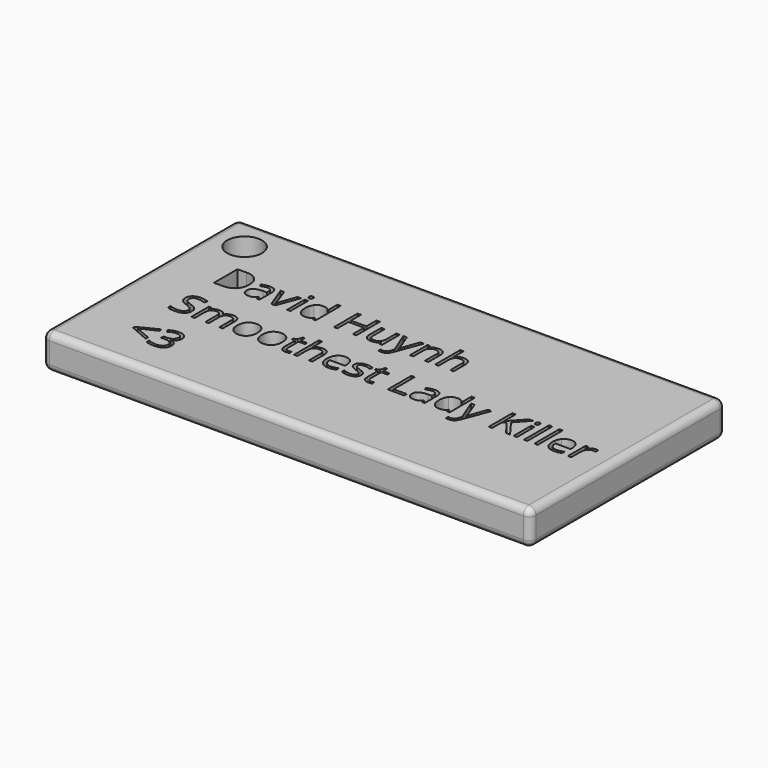
from build123d import *

# Parameters (mm, degrees)
F0_W     = 70
F0_H     = 35
F0_W_2   = 0.4794088215
F0_H_2   = 3.1637287353
F0_H_3   = 4.4920329459
F0_R     = 2.5
F1_DEPTH = 5
F2_R     = 1


with BuildPart() as f1:
    # F0 (on Top) → F1 (new body)
    with BuildSketch(Plane.XY):
        with Locations((35, 17.5)):
            Rectangle(F0_W, F0_H)
        Polygon((10.2831517034, 6.0801306554), (10.2831517034, 5.6441365056), (7.5092312969, 6.8625184624), (7.5092312969, 7.1451756866), (10.2831517034, 8.5279791659), (10.2831517034, 8.0984510311), (8.0255887752, 7.026939985), align=None, mode=Mode.SUBTRACT)
        with BuildLine():
            add(Edge.make_bspline(
                [(13.152214901, 8.9450371291), (13.4930662596, 8.6637654795), (13.4930662596, 8.173272061)],
                knots=[0, 0, 0, 1, 1, 1], degree=2))
            add(Edge.make_bspline(
                [(13.4930662596, 8.173272061), (13.4930662596, 7.7686842695), (13.2662938787, 7.511891105)],
                knots=[0, 0, 0, 1, 1, 1], degree=2))
            add(Edge.make_bspline(
                [(13.2662938787, 7.511891105), (13.0395214978, 7.2550979405), (12.6238491093, 7.1682685971)],
                knots=[0, 0, 0, 1, 1, 1], degree=2))
            Line((12.6238491093, 7.1682685971), (12.6238491093, 7.1451756866))
            add(Edge.make_bspline(
                [(12.6238491093, 7.1451756866), (13.1318931398, 7.0823629701), (13.377139849, 6.8223367981)],
                knots=[0, 0, 0, 1, 1, 1], degree=2))
            add(Edge.make_bspline(
                [(13.377139849, 6.8223367981), (13.6223865583, 6.5623106262), (13.6223865583, 6.1410959391)],
                knots=[0, 0, 0, 1, 1, 1], degree=2))
            add(Edge.make_bspline(
                [(13.6223865583, 6.1410959391), (13.6223865583, 5.5379091174), (13.2039430204, 5.2127609379)],
                knots=[0, 0, 0, 1, 1, 1], degree=2))
            add(Edge.make_bspline(
                [(13.2039430204, 5.2127609379), (12.7854994826, 4.8876127584), (12.0151199891, 4.8876127584)],
                knots=[0, 0, 0, 1, 1, 1], degree=2))
            add(Edge.make_bspline(
                [(12.0151199891, 4.8876127584), (11.679810929, 4.8876127584), (11.4013104286, 4.9384171615)],
                knots=[0, 0, 0, 1, 1, 1], degree=2))
            add(Edge.make_bspline(
                [(11.4013104286, 4.9384171615), (11.1228099283, 4.9892215645), (10.8604744653, 5.1157707139)],
                knots=[0, 0, 0, 1, 1, 1], degree=2))
            Line((10.8604744653, 5.1157707139), (10.8604744653, 5.5720866249))
            add(Edge.make_bspline(
                [(10.8604744653, 5.5720866249), (11.1348182417, 5.4363003113), (11.4451869586, 5.3656360053)],
                knots=[0, 0, 0, 1, 1, 1], degree=2))
            add(Edge.make_bspline(
                [(11.4451869586, 5.3656360053), (11.7555556754, 5.2949716992), (12.0326706011, 5.2949716992)],
                knots=[0, 0, 0, 1, 1, 1], degree=2))
            add(Edge.make_bspline(
                [(12.0326706011, 5.2949716992), (13.1263508412, 5.2949716992), (13.1263508412, 6.1521805361)],
                knots=[0, 0, 0, 1, 1, 1], degree=2))
            add(Edge.make_bspline(
                [(13.1263508412, 6.1521805361), (13.1263508412, 6.9207125968), (11.9199771979, 6.9207125968)],
                knots=[0, 0, 0, 1, 1, 1], degree=2))
            Line((11.9199771979, 6.9207125968), (11.5043048094, 6.9207125968))
            Line((11.5043048094, 6.9207125968), (11.5043048094, 7.3326901197))
            Line((11.5043048094, 7.3326901197), (11.9255194965, 7.3326901197))
            add(Edge.make_bspline(
                [(11.9255194965, 7.3326901197), (12.4187840642, 7.3326901197), (12.7074454452, 7.5506871946)],
                knots=[0, 0, 0, 1, 1, 1], degree=2))
            add(Edge.make_bspline(
                [(12.7074454452, 7.5506871946), (12.9961068262, 7.7686842695), (12.9961068262, 8.1557214491)],
                knots=[0, 0, 0, 1, 1, 1], degree=2))
            add(Edge.make_bspline(
                [(12.9961068262, 8.1557214491), (12.9961068262, 8.464242733), (12.784113908, 8.6406725691)],
                knots=[0, 0, 0, 1, 1, 1], degree=2))
            add(Edge.make_bspline(
                [(12.784113908, 8.6406725691), (12.5721209898, 8.8171024051), (12.2081767207, 8.8171024051)],
                knots=[0, 0, 0, 1, 1, 1], degree=2))
            add(Edge.make_bspline(
                [(12.2081767207, 8.8171024051), (11.931061795, 8.8171024051), (11.6858150857, 8.7418195169)],
                knots=[0, 0, 0, 1, 1, 1], degree=2))
            add(Edge.make_bspline(
                [(11.6858150857, 8.7418195169), (11.4405683765, 8.6665366288), (11.1255810776, 8.464242733)],
                knots=[0, 0, 0, 1, 1, 1], degree=2))
            Line((11.1255810776, 8.464242733), (10.8835673758, 8.7875434797))
            add(Edge.make_bspline(
                [(10.8835673758, 8.7875434797), (11.1431316895, 8.9926085247), (11.4821356153, 9.1094586517)],
                knots=[0, 0, 0, 1, 1, 1], degree=2))
            add(Edge.make_bspline(
                [(11.4821356153, 9.1094586517), (11.8211395411, 9.2263087787), (12.1970921237, 9.2263087787)],
                knots=[0, 0, 0, 1, 1, 1], degree=2))
            add(Edge.make_bspline(
                [(12.1970921237, 9.2263087787), (12.8113635423, 9.2263087787), (13.152214901, 8.9450371291)],
                knots=[0, 0, 0, 1, 1, 1], degree=2))
        make_face(mode=Mode.SUBTRACT)
        with BuildLine():
            add(Edge.make_bspline(
                [(9.9210548671, 14.8129456812), (10.1704583003, 14.541373054), (10.1704583003, 14.1090737699)],
                knots=[0, 0, 0, 1, 1, 1], degree=2))
            add(Edge.make_bspline(
                [(10.1704583003, 14.1090737699), (10.1704583003, 13.5520727692), (9.7663323669, 13.2398566196)],
                knots=[0, 0, 0, 1, 1, 1], degree=2))
            add(Edge.make_bspline(
                [(9.7663323669, 13.2398566196), (9.3622064336, 12.9276404699), (8.6694191193, 12.9276404699)],
                knots=[0, 0, 0, 1, 1, 1], degree=2))
            add(Edge.make_bspline(
                [(8.6694191193, 12.9276404699), (7.919361387, 12.9276404699), (7.5147735955, 13.1216209179)],
                knots=[0, 0, 0, 1, 1, 1], degree=2))
            Line((7.5147735955, 13.1216209179), (7.5147735955, 13.5945637245))
            add(Edge.make_bspline(
                [(7.5147735955, 13.5945637245), (7.7752616256, 13.485565187), (8.0810117603, 13.4218287541)],
                knots=[0, 0, 0, 1, 1, 1], degree=2))
            add(Edge.make_bspline(
                [(8.0810117603, 13.4218287541), (8.386761895, 13.3580923212), (8.6869697312, 13.3580923212)],
                knots=[0, 0, 0, 1, 1, 1], degree=2))
            add(Edge.make_bspline(
                [(8.6869697312, 13.3580923212), (9.1774631498, 13.3580923212), (9.4259428665, 13.5442211796)],
                knots=[0, 0, 0, 1, 1, 1], degree=2))
            add(Edge.make_bspline(
                [(9.4259428665, 13.5442211796), (9.6744225832, 13.7303500381), (9.6744225832, 14.0628879489)],
                knots=[0, 0, 0, 1, 1, 1], degree=2))
            add(Edge.make_bspline(
                [(9.6744225832, 14.0628879489), (9.6744225832, 14.2818087403), (9.5862076652, 14.4217517777)],
                knots=[0, 0, 0, 1, 1, 1], degree=2))
            add(Edge.make_bspline(
                [(9.5862076652, 14.4217517777), (9.4979927472, 14.5616948152), (9.2915421275, 14.6803923751)],
                knots=[0, 0, 0, 1, 1, 1], degree=2))
            add(Edge.make_bspline(
                [(9.2915421275, 14.6803923751), (9.0850915079, 14.7990899349), (8.6638768208, 14.9487319948)],
                knots=[0, 0, 0, 1, 1, 1], degree=2))
            add(Edge.make_bspline(
                [(8.6638768208, 14.9487319948), (8.0754694618, 15.1593393384), (7.8228330212, 15.4480007193)],
                knots=[0, 0, 0, 1, 1, 1], degree=2))
            add(Edge.make_bspline(
                [(7.8228330212, 15.4480007193), (7.5701965806, 15.7366621003), (7.5701965806, 16.2012914591)],
                knots=[0, 0, 0, 1, 1, 1], degree=2))
            add(Edge.make_bspline(
                [(7.5701965806, 16.2012914591), (7.5701965806, 16.6890137283), (7.9364501408, 16.9776751093)],
                knots=[0, 0, 0, 1, 1, 1], degree=2))
            add(Edge.make_bspline(
                [(7.9364501408, 16.9776751093), (8.3027037009, 17.2663364902), (8.906814239, 17.2663364902)],
                knots=[0, 0, 0, 1, 1, 1], degree=2))
            add(Edge.make_bspline(
                [(8.906814239, 17.2663364902), (9.5358651204, 17.2663364902), (10.0642309121, 17.0354073855)],
                knots=[0, 0, 0, 1, 1, 1], degree=2))
            Line((10.0642309121, 17.0354073855), (9.9108939865, 16.6086503999))
            add(Edge.make_bspline(
                [(9.9108939865, 16.6086503999), (9.3880704933, 16.8275711912), (8.8948059255, 16.8275711912)],
                knots=[0, 0, 0, 1, 1, 1], degree=2))
            add(Edge.make_bspline(
                [(8.8948059255, 16.8275711912), (8.5049975967, 16.8275711912), (8.2856149472, 16.6603785193)],
                knots=[0, 0, 0, 1, 1, 1], degree=2))
            add(Edge.make_bspline(
                [(8.2856149472, 16.6603785193), (8.0662322976, 16.4931858475), (8.0662322976, 16.1957491605)],
                knots=[0, 0, 0, 1, 1, 1], degree=2))
            add(Edge.make_bspline(
                [(8.0662322976, 16.1957491605), (8.0662322976, 15.9768283692), (8.1470574843, 15.8364234735)],
                knots=[0, 0, 0, 1, 1, 1], degree=2))
            add(Edge.make_bspline(
                [(8.1470574843, 15.8364234735), (8.227882671, 15.6960185778), (8.4200156861, 15.5791684508)],
                knots=[0, 0, 0, 1, 1, 1], degree=2))
            add(Edge.make_bspline(
                [(8.4200156861, 15.5791684508), (8.6121487013, 15.4623183238), (9.0074993287, 15.3209897117)],
                knots=[0, 0, 0, 1, 1, 1], degree=2))
            add(Edge.make_bspline(
                [(9.0074993287, 15.3209897117), (9.671651434, 15.0845183084), (9.9210548671, 14.8129456812)],
                knots=[0, 0, 0, 1, 1, 1], degree=2))
        make_face(mode=Mode.SUBTRACT)
        with BuildLine():
            Line((15.4735142621, 12.9858346043), (14.995029157, 12.9858346043))
            Line((14.995029157, 12.9858346043), (14.995029157, 15.043874786))
            add(Edge.make_bspline(
                [(14.995029157, 15.043874786), (14.995029157, 15.4225985178), (14.8333787837, 15.6114985255)],
                knots=[0, 0, 0, 1, 1, 1], degree=2))
            add(Edge.make_bspline(
                [(14.8333787837, 15.6114985255), (14.6717284103, 15.8003985332), (14.3308770517, 15.8003985332)],
                knots=[0, 0, 0, 1, 1, 1], degree=2))
            add(Edge.make_bspline(
                [(14.3308770517, 15.8003985332), (13.8837983049, 15.8003985332), (13.6699579539, 15.5436053687)],
                knots=[0, 0, 0, 1, 1, 1], degree=2))
            add(Edge.make_bspline(
                [(13.6699579539, 15.5436053687), (13.4561176028, 15.2868122042), (13.4561176028, 14.752904114)],
                knots=[0, 0, 0, 1, 1, 1], degree=2))
            Line((13.4561176028, 14.752904114), (13.4561176028, 12.9858346043))
            Line((13.4561176028, 12.9858346043), (12.9767087814, 12.9858346043))
            Line((12.9767087814, 12.9858346043), (12.9767087814, 15.043874786))
            add(Edge.make_bspline(
                [(12.9767087814, 15.043874786), (12.9767087814, 15.4225985178), (12.815058408, 15.6114985255)],
                knots=[0, 0, 0, 1, 1, 1], degree=2))
            add(Edge.make_bspline(
                [(12.815058408, 15.6114985255), (12.6534080347, 15.8003985332), (12.3097855268, 15.8003985332)],
                knots=[0, 0, 0, 1, 1, 1], degree=2))
            add(Edge.make_bspline(
                [(12.3097855268, 15.8003985332), (11.8599356307, 15.8003985332), (11.6507138618, 15.5306733388)],
                knots=[0, 0, 0, 1, 1, 1], degree=2))
            add(Edge.make_bspline(
                [(11.6507138618, 15.5306733388), (11.4414920929, 15.2609481445), (11.4414920929, 14.6457530094)],
                knots=[0, 0, 0, 1, 1, 1], degree=2))
            Line((11.4414920929, 14.6457530094), (11.4414920929, 12.9858346043))
            Line((11.4414920929, 12.9858346043), (10.9620832714, 12.9858346043))
            Line((10.9620832714, 12.9858346043), (10.9620832714, 16.1495633396))
            Line((10.9620832714, 16.1495633396), (11.3518916002, 16.1495633396))
            Line((11.3518916002, 16.1495633396), (11.4294837794, 15.7163403391))
            Line((11.4294837794, 15.7163403391), (11.4525766899, 15.7163403391))
            add(Edge.make_bspline(
                [(11.4525766899, 15.7163403391), (11.5883630035, 15.9472694438), (11.8354571456, 16.0775134589)],
                knots=[0, 0, 0, 1, 1, 1], degree=2))
            add(Edge.make_bspline(
                [(11.8354571456, 16.0775134589), (12.0825512877, 16.207757474), (12.3883014224, 16.207757474)],
                knots=[0, 0, 0, 1, 1, 1], degree=2))
            add(Edge.make_bspline(
                [(12.3883014224, 16.207757474), (13.1300457069, 16.207757474), (13.3582036624, 15.6701545181)],
                knots=[0, 0, 0, 1, 1, 1], degree=2))
            Line((13.3582036624, 15.6701545181), (13.3812965729, 15.6701545181))
            add(Edge.make_bspline(
                [(13.3812965729, 15.6701545181), (13.522625185, 15.9186342348), (13.7909648048, 16.0631958544)],
                knots=[0, 0, 0, 1, 1, 1], degree=2))
            add(Edge.make_bspline(
                [(13.7909648048, 16.0631958544), (14.0593044245, 16.207757474), (14.4029269324, 16.207757474)],
                knots=[0, 0, 0, 1, 1, 1], degree=2))
            add(Edge.make_bspline(
                [(14.4029269324, 16.207757474), (14.9396061719, 16.207757474), (15.206560217, 15.9320281229)],
                knots=[0, 0, 0, 1, 1, 1], degree=2))
            add(Edge.make_bspline(
                [(15.206560217, 15.9320281229), (15.4735142621, 15.6562987718), (15.4735142621, 15.0494170845)],
                knots=[0, 0, 0, 1, 1, 1], degree=2))
            Line((15.4735142621, 15.0494170845), (15.4735142621, 12.9858346043))
        make_face(mode=Mode.SUBTRACT)
        with BuildLine():
            add(Edge.make_bspline(
                [(18.8002789453, 15.7657591675), (19.1914728488, 15.323760861), (19.1914728488, 14.5709319794)],
                knots=[0, 0, 0, 1, 1, 1], degree=2))
            add(Edge.make_bspline(
                [(19.1914728488, 14.5709319794), (19.1914728488, 13.7968576202), (18.8021263782, 13.3622490451)],
                knots=[0, 0, 0, 1, 1, 1], degree=2))
            add(Edge.make_bspline(
                [(18.8021263782, 13.3622490451), (18.4127799075, 12.9276404699), (17.7255348917, 12.9276404699)],
                knots=[0, 0, 0, 1, 1, 1], degree=2))
            add(Edge.make_bspline(
                [(17.7255348917, 12.9276404699), (17.300625339, 12.9276404699), (16.9717822938, 13.1271632164)],
                knots=[0, 0, 0, 1, 1, 1], degree=2))
            add(Edge.make_bspline(
                [(16.9717822938, 13.1271632164), (16.6429392486, 13.3266859629), (16.4637382633, 13.6989436798)],
                knots=[0, 0, 0, 1, 1, 1], degree=2))
            add(Edge.make_bspline(
                [(16.4637382633, 13.6989436798), (16.284537278, 14.0712013967), (16.284537278, 14.5709319794)],
                knots=[0, 0, 0, 1, 1, 1], degree=2))
            add(Edge.make_bspline(
                [(16.284537278, 14.5709319794), (16.284537278, 15.3440826222), (16.6715744576, 15.7759200481)],
                knots=[0, 0, 0, 1, 1, 1], degree=2))
            add(Edge.make_bspline(
                [(16.6715744576, 15.7759200481), (17.0586116372, 16.207757474), (17.745856653, 16.207757474)],
                knots=[0, 0, 0, 1, 1, 1], degree=2))
            add(Edge.make_bspline(
                [(17.745856653, 16.207757474), (18.4090850418, 16.207757474), (18.8002789453, 15.7657591675)],
                knots=[0, 0, 0, 1, 1, 1], degree=2))
        make_face(mode=Mode.SUBTRACT)
        with BuildLine():
            add(Edge.make_bspline(
                [(22.3713666214, 15.7657591675), (22.7625605249, 15.323760861), (22.7625605249, 14.5709319794)],
                knots=[0, 0, 0, 1, 1, 1], degree=2))
            add(Edge.make_bspline(
                [(22.7625605249, 14.5709319794), (22.7625605249, 13.7968576202), (22.3732140542, 13.3622490451)],
                knots=[0, 0, 0, 1, 1, 1], degree=2))
            add(Edge.make_bspline(
                [(22.3732140542, 13.3622490451), (21.9838675836, 12.9276404699), (21.2966225678, 12.9276404699)],
                knots=[0, 0, 0, 1, 1, 1], degree=2))
            add(Edge.make_bspline(
                [(21.2966225678, 12.9276404699), (20.8717130151, 12.9276404699), (20.5428699699, 13.1271632164)],
                knots=[0, 0, 0, 1, 1, 1], degree=2))
            add(Edge.make_bspline(
                [(20.5428699699, 13.1271632164), (20.2140269247, 13.3266859629), (20.0348259394, 13.6989436798)],
                knots=[0, 0, 0, 1, 1, 1], degree=2))
            add(Edge.make_bspline(
                [(20.0348259394, 13.6989436798), (19.8556249541, 14.0712013967), (19.8556249541, 14.5709319794)],
                knots=[0, 0, 0, 1, 1, 1], degree=2))
            add(Edge.make_bspline(
                [(19.8556249541, 14.5709319794), (19.8556249541, 15.3440826222), (20.2426621337, 15.7759200481)],
                knots=[0, 0, 0, 1, 1, 1], degree=2))
            add(Edge.make_bspline(
                [(20.2426621337, 15.7759200481), (20.6296993133, 16.207757474), (21.316944329, 16.207757474)],
                knots=[0, 0, 0, 1, 1, 1], degree=2))
            add(Edge.make_bspline(
                [(21.316944329, 16.207757474), (21.9801727179, 16.207757474), (22.3713666214, 15.7657591675)],
                knots=[0, 0, 0, 1, 1, 1], degree=2))
        make_face(mode=Mode.SUBTRACT)
        with BuildLine():
            add(Edge.make_bspline(
                [(24.2525151088, 13.476789881), (24.3883014224, 13.3239148137), (24.6247728257, 13.3239148137)],
                knots=[0, 0, 0, 1, 1, 1], degree=2))
            add(Edge.make_bspline(
                [(24.6247728257, 13.3239148137), (24.7522456915, 13.3239148137), (24.8704813932, 13.3423891421)],
                knots=[0, 0, 0, 1, 1, 1], degree=2))
            add(Edge.make_bspline(
                [(24.8704813932, 13.3423891421), (24.9887170948, 13.3608634705), (25.0579958262, 13.3811852317)],
                knots=[0, 0, 0, 1, 1, 1], degree=2))
            Line((25.0579958262, 13.3811852317), (25.0579958262, 13.0144698133))
            add(Edge.make_bspline(
                [(25.0579958262, 13.0144698133), (24.980403647, 12.9775211565), (24.8289141543, 12.9525808132)],
                knots=[0, 0, 0, 1, 1, 1], degree=2))
            add(Edge.make_bspline(
                [(24.8289141543, 12.9525808132), (24.6774246616, 12.9276404699), (24.5554940943, 12.9276404699)],
                knots=[0, 0, 0, 1, 1, 1], degree=2))
            add(Edge.make_bspline(
                [(24.5554940943, 12.9276404699), (23.6382436901, 12.9276404699), (23.6382436901, 13.8947715607)],
                knots=[0, 0, 0, 1, 1, 1], degree=2))
            Line((23.6382436901, 13.8947715607), (23.6382436901, 15.7773056227))
            Line((23.6382436901, 15.7773056227), (23.1846989284, 15.7773056227))
            Line((23.1846989284, 15.7773056227), (23.1846989284, 16.0082347275))
            Line((23.1846989284, 16.0082347275), (23.6382436901, 16.207757474))
            Line((23.6382436901, 16.207757474), (23.8396138695, 16.8829941763))
            Line((23.8396138695, 16.8829941763), (24.1167287952, 16.8829941763))
            Line((24.1167287952, 16.8829941763), (24.1167287952, 16.1495633396))
            Line((24.1167287952, 16.1495633396), (25.0349029158, 16.1495633396))
            Line((25.0349029158, 16.1495633396), (25.0349029158, 15.7773056227))
            Line((25.0349029158, 15.7773056227), (24.1167287952, 15.7773056227))
            Line((24.1167287952, 15.7773056227), (24.1167287952, 13.9150933219))
            add(Edge.make_bspline(
                [(24.1167287952, 13.9150933219), (24.1167287952, 13.6296649484), (24.2525151088, 13.476789881)],
                knots=[0, 0, 0, 1, 1, 1], degree=2))
        make_face(mode=Mode.SUBTRACT)
        with BuildLine():
            Line((28.3344179646, 12.9858346043), (27.8550091431, 12.9858346043))
            Line((27.8550091431, 12.9858346043), (27.8550091431, 15.0327901889))
            add(Edge.make_bspline(
                [(27.8550091431, 15.0327901889), (27.8550091431, 15.4189036521), (27.6790411653, 15.6096510927)],
                knots=[0, 0, 0, 1, 1, 1], degree=2))
            add(Edge.make_bspline(
                [(27.6790411653, 15.6096510927), (27.5030731875, 15.8003985332), (27.1271206049, 15.8003985332)],
                knots=[0, 0, 0, 1, 1, 1], degree=2))
            add(Edge.make_bspline(
                [(27.1271206049, 15.8003985332), (26.6283137386, 15.8003985332), (26.3987702085, 15.528825906)],
                knots=[0, 0, 0, 1, 1, 1], degree=2))
            add(Edge.make_bspline(
                [(26.3987702085, 15.528825906), (26.1692266784, 15.2572532788), (26.1692266784, 14.6402107108)],
                knots=[0, 0, 0, 1, 1, 1], degree=2))
            Line((26.1692266784, 14.6402107108), (26.1692266784, 12.9858346043))
            Line((26.1692266784, 12.9858346043), (25.6898178569, 12.9858346043))
            Line((25.6898178569, 12.9858346043), (25.6898178569, 17.4778675502))
            Line((25.6898178569, 17.4778675502), (26.1692266784, 17.4778675502))
            Line((26.1692266784, 17.4778675502), (26.1692266784, 16.1181569813))
            add(Edge.make_bspline(
                [(26.1692266784, 16.1181569813), (26.1692266784, 15.8724484139), (26.1461337679, 15.7107980405)],
                knots=[0, 0, 0, 1, 1, 1], degree=2))
            Line((26.1461337679, 15.7107980405), (26.1747689769, 15.7107980405))
            add(Edge.make_bspline(
                [(26.1747689769, 15.7107980405), (26.316097589, 15.938955996), (26.5775093356, 16.0701237276)],
                knots=[0, 0, 0, 1, 1, 1], degree=2))
            add(Edge.make_bspline(
                [(26.5775093356, 16.0701237276), (26.8389210822, 16.2012914591), (27.1733064259, 16.2012914591)],
                knots=[0, 0, 0, 1, 1, 1], degree=2))
            add(Edge.make_bspline(
                [(27.1733064259, 16.2012914591), (27.753400337, 16.2012914591), (28.0439091508, 15.925562108)],
                knots=[0, 0, 0, 1, 1, 1], degree=2))
            add(Edge.make_bspline(
                [(28.0439091508, 15.925562108), (28.3344179646, 15.6498327569), (28.3344179646, 15.0494170845)],
                knots=[0, 0, 0, 1, 1, 1], degree=2))
            Line((28.3344179646, 15.0494170845), (28.3344179646, 12.9858346043))
        make_face(mode=Mode.SUBTRACT)
        with BuildLine():
            add(Edge.make_bspline(
                [(31.2016337294, 12.9756737237), (30.9753232067, 12.9276404699), (30.6547936093, 12.9276404699)],
                knots=[0, 0, 0, 1, 1, 1], degree=2))
            add(Edge.make_bspline(
                [(30.6547936093, 12.9276404699), (29.9536928472, 12.9276404699), (29.5477194811, 13.3553211719)],
                knots=[0, 0, 0, 1, 1, 1], degree=2))
            add(Edge.make_bspline(
                [(29.5477194811, 13.3553211719), (29.1417461149, 13.783001874), (29.1417461149, 14.541373054)],
                knots=[0, 0, 0, 1, 1, 1], degree=2))
            add(Edge.make_bspline(
                [(29.1417461149, 14.541373054), (29.1417461149, 15.3071339654), (29.5186224139, 15.7574457197)],
                knots=[0, 0, 0, 1, 1, 1], degree=2))
            add(Edge.make_bspline(
                [(29.5186224139, 15.7574457197), (29.8954987128, 16.207757474), (30.5310156092, 16.207757474)],
                knots=[0, 0, 0, 1, 1, 1], degree=2))
            add(Edge.make_bspline(
                [(30.5310156092, 16.207757474), (31.1249652666, 16.207757474), (31.4713589238, 15.8165635705)],
                knots=[0, 0, 0, 1, 1, 1], degree=2))
            add(Edge.make_bspline(
                [(31.4713589238, 15.8165635705), (31.8177525809, 15.425369667), (31.8177525809, 14.7843104722)],
                knots=[0, 0, 0, 1, 1, 1], degree=2))
            Line((31.8177525809, 14.7843104722), (31.8177525809, 14.4813314868))
            Line((31.8177525809, 14.4813314868), (29.6387055483, 14.4813314868))
            add(Edge.make_bspline(
                [(29.6387055483, 14.4813314868), (29.653485011, 13.9243304861), (29.9204390562, 13.6356691051)],
                knots=[0, 0, 0, 1, 1, 1], degree=2))
            add(Edge.make_bspline(
                [(29.9204390562, 13.6356691051), (30.1873931013, 13.3470077242), (30.6723442213, 13.3470077242)],
                knots=[0, 0, 0, 1, 1, 1], degree=2))
            add(Edge.make_bspline(
                [(30.6723442213, 13.3470077242), (31.183159401, 13.3470077242), (31.6819662673, 13.560386217)],
                knots=[0, 0, 0, 1, 1, 1], degree=2))
            Line((31.6819662673, 13.560386217), (31.6819662673, 13.1327055149))
            add(Edge.make_bspline(
                [(31.6819662673, 13.1327055149), (31.4279442521, 13.0237069775), (31.2016337294, 12.9756737237)],
                knots=[0, 0, 0, 1, 1, 1], degree=2))
        make_face(mode=Mode.SUBTRACT)
        with BuildLine():
            add(Edge.make_bspline(
                [(34.4780558678, 14.3714092329), (34.6757311815, 14.1635730386), (34.6757311815, 13.8485857397)],
                knots=[0, 0, 0, 1, 1, 1], degree=2))
            add(Edge.make_bspline(
                [(34.6757311815, 13.8485857397), (34.6757311815, 13.4070492914), (34.3468881363, 13.1673448807)],
                knots=[0, 0, 0, 1, 1, 1], degree=2))
            add(Edge.make_bspline(
                [(34.3468881363, 13.1673448807), (34.0180450911, 12.9276404699), (33.4231717172, 12.9276404699)],
                knots=[0, 0, 0, 1, 1, 1], degree=2))
            add(Edge.make_bspline(
                [(33.4231717172, 12.9276404699), (32.7941208359, 12.9276404699), (32.4421848802, 13.1271632164)],
                knots=[0, 0, 0, 1, 1, 1], degree=2))
            Line((32.4421848802, 13.1271632164), (32.4421848802, 13.571470814))
            add(Edge.make_bspline(
                [(32.4421848802, 13.571470814), (32.6703428357, 13.4560062616), (32.9312927241, 13.3899605377)],
                knots=[0, 0, 0, 1, 1, 1], degree=2))
            add(Edge.make_bspline(
                [(32.9312927241, 13.3899605377), (33.1922426125, 13.3239148137), (33.4351800307, 13.3239148137)],
                knots=[0, 0, 0, 1, 1, 1], degree=2))
            add(Edge.make_bspline(
                [(33.4351800307, 13.3239148137), (33.8102088968, 13.3239148137), (34.0120409344, 13.44353609)],
                knots=[0, 0, 0, 1, 1, 1], degree=2))
            add(Edge.make_bspline(
                [(34.0120409344, 13.44353609), (34.2138729719, 13.5631573662), (34.2138729719, 13.8088659337)],
                knots=[0, 0, 0, 1, 1, 1], degree=2))
            add(Edge.make_bspline(
                [(34.2138729719, 13.8088659337), (34.2138729719, 13.9936092175), (34.0540700314, 14.124776949)],
                knots=[0, 0, 0, 1, 1, 1], degree=2))
            add(Edge.make_bspline(
                [(34.0540700314, 14.124776949), (33.894267091, 14.2559446805), (33.4287140157, 14.4351456658)],
                knots=[0, 0, 0, 1, 1, 1], degree=2))
            add(Edge.make_bspline(
                [(33.4287140157, 14.4351456658), (32.9871775674, 14.5995671884), (32.801048709, 14.7224214721)],
                knots=[0, 0, 0, 1, 1, 1], degree=2))
            add(Edge.make_bspline(
                [(32.801048709, 14.7224214721), (32.6149198506, 14.8452757559), (32.5239337833, 15.0009219725)],
                knots=[0, 0, 0, 1, 1, 1], degree=2))
            add(Edge.make_bspline(
                [(32.5239337833, 15.0009219725), (32.432947716, 15.1565681891), (32.432947716, 15.3727178312)],
                knots=[0, 0, 0, 1, 1, 1], degree=2))
            add(Edge.make_bspline(
                [(32.432947716, 15.3727178312), (32.432947716, 15.7597550107), (32.7479350149, 15.9837562424)],
                knots=[0, 0, 0, 1, 1, 1], degree=2))
            add(Edge.make_bspline(
                [(32.7479350149, 15.9837562424), (33.0629223138, 16.207757474), (33.6106861503, 16.207757474)],
                knots=[0, 0, 0, 1, 1, 1], degree=2))
            add(Edge.make_bspline(
                [(33.6106861503, 16.207757474), (34.12150133, 16.207757474), (34.6101473157, 15.9999212797)],
                knots=[0, 0, 0, 1, 1, 1], degree=2))
            Line((34.6101473157, 15.9999212797), (34.4392597782, 15.6101129509))
            add(Edge.make_bspline(
                [(34.4392597782, 15.6101129509), (33.9635458224, 15.8059408317), (33.5765086428, 15.8059408317)],
                knots=[0, 0, 0, 1, 1, 1], degree=2))
            add(Edge.make_bspline(
                [(33.5765086428, 15.8059408317), (33.2356572842, 15.8059408317), (33.0624604556, 15.6992515853)],
                knots=[0, 0, 0, 1, 1, 1], degree=2))
            add(Edge.make_bspline(
                [(33.0624604556, 15.6992515853), (32.889263627, 15.5925623389), (32.889263627, 15.4050479058)],
                knots=[0, 0, 0, 1, 1, 1], degree=2))
            add(Edge.make_bspline(
                [(32.889263627, 15.4050479058), (32.889263627, 15.27757504), (32.9543856346, 15.1884364056)],
                knots=[0, 0, 0, 1, 1, 1], degree=2))
            add(Edge.make_bspline(
                [(32.9543856346, 15.1884364056), (33.0195076421, 15.0992977711), (33.1636074035, 15.0184725845)],
                knots=[0, 0, 0, 1, 1, 1], degree=2))
            add(Edge.make_bspline(
                [(33.1636074035, 15.0184725845), (33.3077071648, 14.9376473978), (33.7178372549, 14.7843104722)],
                knots=[0, 0, 0, 1, 1, 1], degree=2))
            add(Edge.make_bspline(
                [(33.7178372549, 14.7843104722), (34.2803805541, 14.5792454272), (34.4780558678, 14.3714092329)],
                knots=[0, 0, 0, 1, 1, 1], degree=2))
        make_face(mode=Mode.SUBTRACT)
        with BuildLine():
            add(Edge.make_bspline(
                [(36.1047204818, 13.476789881), (36.2405067954, 13.3239148137), (36.4769781986, 13.3239148137)],
                knots=[0, 0, 0, 1, 1, 1], degree=2))
            add(Edge.make_bspline(
                [(36.4769781986, 13.3239148137), (36.6044510645, 13.3239148137), (36.7226867661, 13.3423891421)],
                knots=[0, 0, 0, 1, 1, 1], degree=2))
            add(Edge.make_bspline(
                [(36.7226867661, 13.3423891421), (36.8409224678, 13.3608634705), (36.9102011992, 13.3811852317)],
                knots=[0, 0, 0, 1, 1, 1], degree=2))
            Line((36.9102011992, 13.3811852317), (36.9102011992, 13.0144698133))
            add(Edge.make_bspline(
                [(36.9102011992, 13.0144698133), (36.83260902, 12.9775211565), (36.6811195273, 12.9525808132)],
                knots=[0, 0, 0, 1, 1, 1], degree=2))
            add(Edge.make_bspline(
                [(36.6811195273, 12.9525808132), (36.5296300345, 12.9276404699), (36.4076994672, 12.9276404699)],
                knots=[0, 0, 0, 1, 1, 1], degree=2))
            add(Edge.make_bspline(
                [(36.4076994672, 12.9276404699), (35.4904490631, 12.9276404699), (35.4904490631, 13.8947715607)],
                knots=[0, 0, 0, 1, 1, 1], degree=2))
            Line((35.4904490631, 13.8947715607), (35.4904490631, 15.7773056227))
            Line((35.4904490631, 15.7773056227), (35.0369043013, 15.7773056227))
            Line((35.0369043013, 15.7773056227), (35.0369043013, 16.0082347275))
            Line((35.0369043013, 16.0082347275), (35.4904490631, 16.207757474))
            Line((35.4904490631, 16.207757474), (35.6918192424, 16.8829941763))
            Line((35.6918192424, 16.8829941763), (35.9689341682, 16.8829941763))
            Line((35.9689341682, 16.8829941763), (35.9689341682, 16.1495633396))
            Line((35.9689341682, 16.1495633396), (36.8871082887, 16.1495633396))
            Line((36.8871082887, 16.1495633396), (36.8871082887, 15.7773056227))
            Line((36.8871082887, 15.7773056227), (35.9689341682, 15.7773056227))
            Line((35.9689341682, 15.7773056227), (35.9689341682, 13.9150933219))
            add(Edge.make_bspline(
                [(35.9689341682, 13.9150933219), (35.9689341682, 13.6296649484), (36.1047204818, 13.476789881)],
                knots=[0, 0, 0, 1, 1, 1], degree=2))
        make_face(mode=Mode.SUBTRACT)
        Polygon((41.5029192347, 12.9858346043), (39.1502135154, 12.9858346043), (39.1502135154, 17.206294923), (39.6407069339, 17.206294923), (39.6407069339, 13.4301422019), (41.5029192347, 13.4301422019), align=None, mode=Mode.SUBTRACT)
        with BuildLine():
            Line((44.4477271787, 12.9858346043), (44.0920963574, 12.9858346043))
            Line((44.0920963574, 12.9858346043), (43.9969535662, 13.4366082168))
            Line((43.9969535662, 13.4366082168), (43.9738606557, 13.4366082168))
            add(Edge.make_bspline(
                [(43.9738606557, 13.4366082168), (43.7373892524, 13.1391715299), (43.5023034238, 13.0334059999)],
                knots=[0, 0, 0, 1, 1, 1], degree=2))
            add(Edge.make_bspline(
                [(43.5023034238, 13.0334059999), (43.2672175951, 12.9276404699), (42.9143579231, 12.9276404699)],
                knots=[0, 0, 0, 1, 1, 1], degree=2))
            add(Edge.make_bspline(
                [(42.9143579231, 12.9276404699), (42.4441862658, 12.9276404699), (42.1772322207, 13.1705778881)],
                knots=[0, 0, 0, 1, 1, 1], degree=2))
            add(Edge.make_bspline(
                [(42.1772322207, 13.1705778881), (41.9102781755, 13.4135153063), (41.9102781755, 13.8605940532)],
                knots=[0, 0, 0, 1, 1, 1], degree=2))
            add(Edge.make_bspline(
                [(41.9102781755, 13.8605940532), (41.9102781755, 14.8184879797), (43.4427237148, 14.8646738007)],
                knots=[0, 0, 0, 1, 1, 1], degree=2))
            Line((43.4427237148, 14.8646738007), (43.9794029542, 14.8822244126))
            Line((43.9794029542, 14.8822244126), (43.9794029542, 15.0789760099))
            add(Edge.make_bspline(
                [(43.9794029542, 15.0789760099), (43.9794029542, 15.4512337268), (43.8196000137, 15.6285872792)],
                knots=[0, 0, 0, 1, 1, 1], degree=2))
            add(Edge.make_bspline(
                [(43.8196000137, 15.6285872792), (43.6597970732, 15.8059408317), (43.3069374012, 15.8059408317)],
                knots=[0, 0, 0, 1, 1, 1], degree=2))
            add(Edge.make_bspline(
                [(43.3069374012, 15.8059408317), (42.9115867738, 15.8059408317), (42.4127799075, 15.5639271299)],
                knots=[0, 0, 0, 1, 1, 1], degree=2))
            Line((42.4127799075, 15.5639271299), (42.2649852805, 15.9306425483))
            add(Edge.make_bspline(
                [(42.2649852805, 15.9306425483), (42.4986855345, 16.0571916977), (42.7771860348, 16.1292415784)],
                knots=[0, 0, 0, 1, 1, 1], degree=2))
            add(Edge.make_bspline(
                [(42.7771860348, 16.1292415784), (43.0556865352, 16.2012914591), (43.3364963266, 16.2012914591)],
                knots=[0, 0, 0, 1, 1, 1], degree=2))
            add(Edge.make_bspline(
                [(43.3364963266, 16.2012914591), (43.901810775, 16.2012914591), (44.1747689769, 15.9505024513)],
                knots=[0, 0, 0, 1, 1, 1], degree=2))
            add(Edge.make_bspline(
                [(44.1747689769, 15.9505024513), (44.4477271787, 15.6997134435), (44.4477271787, 15.1454835921)],
                knots=[0, 0, 0, 1, 1, 1], degree=2))
            Line((44.4477271787, 15.1454835921), (44.4477271787, 12.9858346043))
        make_face(mode=Mode.SUBTRACT)
        with BuildLine():
            Line((47.65117572, 12.9858346043), (47.5874392871, 13.4098204407))
            Line((47.5874392871, 13.4098204407), (47.5615752274, 13.4098204407))
            add(Edge.make_bspline(
                [(47.5615752274, 13.4098204407), (47.2299610329, 12.9276404699), (46.5685800769, 12.9276404699)],
                knots=[0, 0, 0, 1, 1, 1], degree=2))
            add(Edge.make_bspline(
                [(46.5685800769, 12.9276404699), (45.9478426433, 12.9276404699), (45.6028345607, 13.3520881645)],
                knots=[0, 0, 0, 1, 1, 1], degree=2))
            add(Edge.make_bspline(
                [(45.6028345607, 13.3520881645), (45.2578264782, 13.776535859), (45.2578264782, 14.558923666)],
                knots=[0, 0, 0, 1, 1, 1], degree=2))
            add(Edge.make_bspline(
                [(45.2578264782, 14.558923666), (45.2578264782, 15.3413114729), (45.6042201354, 15.7745344735)],
                knots=[0, 0, 0, 1, 1, 1], degree=2))
            add(Edge.make_bspline(
                [(45.6042201354, 15.7745344735), (45.9506137925, 16.207757474), (46.5685800769, 16.207757474)],
                knots=[0, 0, 0, 1, 1, 1], degree=2))
            add(Edge.make_bspline(
                [(46.5685800769, 16.207757474), (47.2124104209, 16.207757474), (47.5560329288, 15.7394332495)],
                knots=[0, 0, 0, 1, 1, 1], degree=2))
            Line((47.5560329288, 15.7394332495), (47.593905302, 15.7394332495))
            Line((47.593905302, 15.7394332495), (47.5735835408, 15.967591205))
            Line((47.5735835408, 15.967591205), (47.5615752274, 16.190206862))
            Line((47.5615752274, 16.190206862), (47.5615752274, 17.4778675502))
            Line((47.5615752274, 17.4778675502), (48.0409840488, 17.4778675502))
            Line((48.0409840488, 17.4778675502), (48.0409840488, 12.9858346043))
            Line((48.0409840488, 12.9858346043), (47.65117572, 12.9858346043))
        make_face(mode=Mode.SUBTRACT)
        with BuildLine():
            Line((49.831146469, 12.9682839923), (48.5545703778, 16.1495633396))
            Line((48.5545703778, 16.1495633396), (49.0690804233, 16.1495633396))
            Line((49.0690804233, 16.1495633396), (49.7618677376, 14.3455451732))
            add(Edge.make_bspline(
                [(49.7618677376, 14.3455451732), (49.9891019766, 13.7275788888), (50.0445249618, 13.4532351124)],
                knots=[0, 0, 0, 1, 1, 1], degree=2))
            Line((50.0445249618, 13.4532351124), (50.0676178723, 13.4532351124))
            add(Edge.make_bspline(
                [(50.0676178723, 13.4532351124), (50.104566529, 13.6010297394), (50.2246496635, 13.9575842772)],
                knots=[0, 0, 0, 1, 1, 1], degree=2))
            add(Edge.make_bspline(
                [(50.2246496635, 13.9575842772), (50.344732798, 14.3141388149), (51.0088849033, 16.1495633396)],
                knots=[0, 0, 0, 1, 1, 1], degree=2))
            Line((51.0088849033, 16.1495633396), (51.5224712323, 16.1495633396))
            Line((51.5224712323, 16.1495633396), (50.1627606634, 12.5470693053))
            add(Edge.make_bspline(
                [(50.1627606634, 12.5470693053), (49.9604667677, 12.013161215), (49.6907415733, 11.7891599834)],
                knots=[0, 0, 0, 1, 1, 1], degree=2))
            add(Edge.make_bspline(
                [(49.6907415733, 11.7891599834), (49.4210163789, 11.5651587518), (49.0284369008, 11.5651587518)],
                knots=[0, 0, 0, 1, 1, 1], degree=2))
            add(Edge.make_bspline(
                [(49.0284369008, 11.5651587518), (48.8085923931, 11.5651587518), (48.5952139003, 11.6150394384)],
                knots=[0, 0, 0, 1, 1, 1], degree=2))
            Line((48.5952139003, 11.6150394384), (48.5952139003, 11.9983817523))
            add(Edge.make_bspline(
                [(48.5952139003, 11.9983817523), (48.7540931244, 11.9642042448), (48.9499210052, 11.9642042448)],
                knots=[0, 0, 0, 1, 1, 1], degree=2))
            add(Edge.make_bspline(
                [(48.9499210052, 11.9642042448), (49.4441092894, 11.9642042448), (49.6547166329, 12.5184340963)],
                knots=[0, 0, 0, 1, 1, 1], degree=2))
            Line((49.6547166329, 12.5184340963), (49.831146469, 12.9682839923))
        make_face(mode=Mode.SUBTRACT)
        Polygon((54.931908535, 15.3727178312), (56.6925120298, 12.9858346043), (56.1151892678, 12.9858346043), (54.5772014301, 15.0327901889), (54.1347412654, 14.6402107108), (54.1347412654, 12.9858346043), (53.6442478469, 12.9858346043), (53.6442478469, 17.206294923), (54.1347412654, 17.206294923), (54.1347412654, 15.1131535174), (56.0486816857, 17.206294923), (56.6287755968, 17.206294923), align=None, mode=Mode.SUBTRACT)
        with Locations((57.440260471, 14.567698972)):
            Rectangle(F0_W_2, F0_H_2, mode=Mode.SUBTRACT)
        with Locations((58.9357573534, 15.2318510773)):
            Rectangle(F0_W_2, F0_H_3, mode=Mode.SUBTRACT)
        with Locations((60.4312542359, 15.2318510773)):
            Rectangle(F0_W_2, F0_H_3, mode=Mode.SUBTRACT)
        with BuildLine():
            add(Edge.make_bspline(
                [(57.2407377245, 16.7656821911), (57.1599125378, 16.8451218031), (57.1599125378, 17.0067721765)],
                knots=[0, 0, 0, 1, 1, 1], degree=2))
            add(Edge.make_bspline(
                [(57.1599125378, 17.0067721765), (57.1599125378, 17.1711936991), (57.2407377245, 17.2478621619)],
                knots=[0, 0, 0, 1, 1, 1], degree=2))
            add(Edge.make_bspline(
                [(57.2407377245, 17.2478621619), (57.3215629111, 17.3245306246), (57.4434934785, 17.3245306246)],
                knots=[0, 0, 0, 1, 1, 1], degree=2))
            add(Edge.make_bspline(
                [(57.4434934785, 17.3245306246), (57.5589580308, 17.3245306246), (57.6425543668, 17.2464765872)],
                knots=[0, 0, 0, 1, 1, 1], degree=2))
            add(Edge.make_bspline(
                [(57.6425543668, 17.2464765872), (57.7261507027, 17.1684225498), (57.7261507027, 17.0067721765)],
                knots=[0, 0, 0, 1, 1, 1], degree=2))
            add(Edge.make_bspline(
                [(57.7261507027, 17.0067721765), (57.7261507027, 16.8451218031), (57.6425543668, 16.7656821911)],
                knots=[0, 0, 0, 1, 1, 1], degree=2))
            add(Edge.make_bspline(
                [(57.6425543668, 16.7656821911), (57.5589580308, 16.6862425791), (57.4434934785, 16.6862425791)],
                knots=[0, 0, 0, 1, 1, 1], degree=2))
            add(Edge.make_bspline(
                [(57.4434934785, 16.6862425791), (57.3215629111, 16.6862425791), (57.2407377245, 16.7656821911)],
                knots=[0, 0, 0, 1, 1, 1], degree=2))
        make_face(mode=Mode.SUBTRACT)
        with BuildLine():
            add(Edge.make_bspline(
                [(63.5705044861, 12.9756737237), (63.3441939634, 12.9276404699), (63.023664366, 12.9276404699)],
                knots=[0, 0, 0, 1, 1, 1], degree=2))
            add(Edge.make_bspline(
                [(63.023664366, 12.9276404699), (62.3225636039, 12.9276404699), (61.9165902377, 13.3553211719)],
                knots=[0, 0, 0, 1, 1, 1], degree=2))
            add(Edge.make_bspline(
                [(61.9165902377, 13.3553211719), (61.5106168716, 13.783001874), (61.5106168716, 14.541373054)],
                knots=[0, 0, 0, 1, 1, 1], degree=2))
            add(Edge.make_bspline(
                [(61.5106168716, 14.541373054), (61.5106168716, 15.3071339654), (61.8874931705, 15.7574457197)],
                knots=[0, 0, 0, 1, 1, 1], degree=2))
            add(Edge.make_bspline(
                [(61.8874931705, 15.7574457197), (62.2643694695, 16.207757474), (62.8998863658, 16.207757474)],
                knots=[0, 0, 0, 1, 1, 1], degree=2))
            add(Edge.make_bspline(
                [(62.8998863658, 16.207757474), (63.4938360233, 16.207757474), (63.8402296804, 15.8165635705)],
                knots=[0, 0, 0, 1, 1, 1], degree=2))
            add(Edge.make_bspline(
                [(63.8402296804, 15.8165635705), (64.1866233376, 15.425369667), (64.1866233376, 14.7843104722)],
                knots=[0, 0, 0, 1, 1, 1], degree=2))
            Line((64.1866233376, 14.7843104722), (64.1866233376, 14.4813314868))
            Line((64.1866233376, 14.4813314868), (62.007576305, 14.4813314868))
            add(Edge.make_bspline(
                [(62.007576305, 14.4813314868), (62.0223557677, 13.9243304861), (62.2893098128, 13.6356691051)],
                knots=[0, 0, 0, 1, 1, 1], degree=2))
            add(Edge.make_bspline(
                [(62.2893098128, 13.6356691051), (62.5562638579, 13.3470077242), (63.041214978, 13.3470077242)],
                knots=[0, 0, 0, 1, 1, 1], degree=2))
            add(Edge.make_bspline(
                [(63.041214978, 13.3470077242), (63.5520301577, 13.3470077242), (64.050837024, 13.560386217)],
                knots=[0, 0, 0, 1, 1, 1], degree=2))
            Line((64.050837024, 13.560386217), (64.050837024, 13.1327055149))
            add(Edge.make_bspline(
                [(64.050837024, 13.1327055149), (63.7968150087, 13.0237069775), (63.5705044861, 12.9756737237)],
                knots=[0, 0, 0, 1, 1, 1], degree=2))
        make_face(mode=Mode.SUBTRACT)
        with BuildLine():
            add(Edge.make_bspline(
                [(65.9019647278, 16.0401029439), (66.1504444445, 16.207757474), (66.4478811314, 16.207757474)],
                knots=[0, 0, 0, 1, 1, 1], degree=2))
            add(Edge.make_bspline(
                [(66.4478811314, 16.207757474), (66.658488475, 16.207757474), (66.8256811468, 16.1726562501)],
                knots=[0, 0, 0, 1, 1, 1], degree=2))
            Line((66.8256811468, 16.1726562501), (66.7591735647, 15.7283486525))
            add(Edge.make_bspline(
                [(66.7591735647, 15.7283486525), (66.5633456838, 15.7717633242), (66.4127799075, 15.7717633242)],
                knots=[0, 0, 0, 1, 1, 1], degree=2))
            add(Edge.make_bspline(
                [(66.4127799075, 15.7717633242), (66.0285138772, 15.7717633242), (65.7560175336, 15.4600090328)],
                knots=[0, 0, 0, 1, 1, 1], degree=2))
            add(Edge.make_bspline(
                [(65.7560175336, 15.4600090328), (65.4835211899, 15.1482547413), (65.4835211899, 14.6836253825)],
                knots=[0, 0, 0, 1, 1, 1], degree=2))
            Line((65.4835211899, 14.6836253825), (65.4835211899, 12.9858346043))
            Line((65.4835211899, 12.9858346043), (65.0041123685, 12.9858346043))
            Line((65.0041123685, 12.9858346043), (65.0041123685, 16.1495633396))
            Line((65.0041123685, 16.1495633396), (65.3994629958, 16.1495633396))
            Line((65.3994629958, 16.1495633396), (65.454885981, 15.5639271299))
            Line((65.454885981, 15.5639271299), (65.4779788914, 15.5639271299))
            add(Edge.make_bspline(
                [(65.4779788914, 15.5639271299), (65.653485011, 15.8724484139), (65.9019647278, 16.0401029439)],
                knots=[0, 0, 0, 1, 1, 1], degree=2))
        make_face(mode=Mode.SUBTRACT)
        with BuildLine():
            Line((14.3281059024, 21.0258623158), (13.9724750811, 21.0258623158))
            Line((13.9724750811, 21.0258623158), (13.8773322899, 21.4766359283))
            Line((13.8773322899, 21.4766359283), (13.8542393795, 21.4766359283))
            add(Edge.make_bspline(
                [(13.8542393795, 21.4766359283), (13.6177679762, 21.1791992414), (13.3826821475, 21.0734337114)],
                knots=[0, 0, 0, 1, 1, 1], degree=2))
            add(Edge.make_bspline(
                [(13.3826821475, 21.0734337114), (13.1475963189, 20.9676681814), (12.7947366468, 20.9676681814)],
                knots=[0, 0, 0, 1, 1, 1], degree=2))
            add(Edge.make_bspline(
                [(12.7947366468, 20.9676681814), (12.3245649895, 20.9676681814), (12.0576109444, 21.2106055996)],
                knots=[0, 0, 0, 1, 1, 1], degree=2))
            add(Edge.make_bspline(
                [(12.0576109444, 21.2106055996), (11.7906568993, 21.4535430178), (11.7906568993, 21.9006217647)],
                knots=[0, 0, 0, 1, 1, 1], degree=2))
            add(Edge.make_bspline(
                [(11.7906568993, 21.9006217647), (11.7906568993, 22.8585156912), (13.3231024385, 22.9047015122)],
                knots=[0, 0, 0, 1, 1, 1], degree=2))
            Line((13.3231024385, 22.9047015122), (13.859781678, 22.9222521241))
            Line((13.859781678, 22.9222521241), (13.859781678, 23.1190037214))
            add(Edge.make_bspline(
                [(13.859781678, 23.1190037214), (13.859781678, 23.4912614383), (13.6999787375, 23.6686149907)],
                knots=[0, 0, 0, 1, 1, 1], degree=2))
            add(Edge.make_bspline(
                [(13.6999787375, 23.6686149907), (13.540175797, 23.8459685432), (13.1873161249, 23.8459685432)],
                knots=[0, 0, 0, 1, 1, 1], degree=2))
            add(Edge.make_bspline(
                [(13.1873161249, 23.8459685432), (12.7919654975, 23.8459685432), (12.2931586312, 23.6039548414)],
                knots=[0, 0, 0, 1, 1, 1], degree=2))
            Line((12.2931586312, 23.6039548414), (12.1453640042, 23.9706702598))
            add(Edge.make_bspline(
                [(12.1453640042, 23.9706702598), (12.3790642582, 24.0972194092), (12.6575647586, 24.1692692899)],
                knots=[0, 0, 0, 1, 1, 1], degree=2))
            add(Edge.make_bspline(
                [(12.6575647586, 24.1692692899), (12.9360652589, 24.2413191706), (13.2168750503, 24.2413191706)],
                knots=[0, 0, 0, 1, 1, 1], degree=2))
            add(Edge.make_bspline(
                [(13.2168750503, 24.2413191706), (13.7821894988, 24.2413191706), (14.0551477006, 23.9905301628)],
                knots=[0, 0, 0, 1, 1, 1], degree=2))
            add(Edge.make_bspline(
                [(14.0551477006, 23.9905301628), (14.3281059024, 23.739741155), (14.3281059024, 23.1855113036)],
                knots=[0, 0, 0, 1, 1, 1], degree=2))
            Line((14.3281059024, 23.1855113036), (14.3281059024, 21.0258623158))
        make_face(mode=Mode.SUBTRACT)
        with BuildLine():
            add(Edge.make_bspline(
                [(10.6124566068, 24.700868089), (11.1579111522, 24.1554135436), (11.1579111522, 23.1762741394)],
                knots=[0, 0, 0, 1, 1, 1], degree=2))
            add(Edge.make_bspline(
                [(11.1579111522, 23.1762741394), (11.1579111522, 22.1315508694), (10.5907492709, 21.5787065926)],
                knots=[0, 0, 0, 1, 1, 1], degree=2))
            add(Edge.make_bspline(
                [(10.5907492709, 21.5787065926), (10.0235873896, 21.0258623158), (8.9585423584, 21.0258623158)],
                knots=[0, 0, 0, 1, 1, 1], degree=2))
            Line((8.9585423584, 21.0258623158), (7.7891173719, 21.0258623158))
            Line((7.7891173719, 21.0258623158), (7.7891173719, 25.2463226345))
            Line((7.7891173719, 25.2463226345), (9.0823203586, 25.2463226345))
            add(Edge.make_bspline(
                [(9.0823203586, 25.2463226345), (10.0670020613, 25.2463226345), (10.6124566068, 24.700868089)],
                knots=[0, 0, 0, 1, 1, 1], degree=2))
        make_face(mode=Mode.SUBTRACT)
        with BuildLine():
            Line((16.5671945022, 21.0258623158), (16.0074223523, 21.0258623158))
            Line((16.0074223523, 21.0258623158), (14.8065910075, 24.1895910511))
            Line((14.8065910075, 24.1895910511), (15.3201773365, 24.1895910511))
            Line((15.3201773365, 24.1895910511), (16.0018800538, 22.313523004))
            add(Edge.make_bspline(
                [(16.0018800538, 22.313523004), (16.2328091585, 21.6549131972), (16.273452681, 21.4590853163)],
                knots=[0, 0, 0, 1, 1, 1], degree=2))
            Line((16.273452681, 21.4590853163), (16.2965455915, 21.4590853163))
            add(Edge.make_bspline(
                [(16.2965455915, 21.4590853163), (16.3279519497, 21.6114985255), (16.4969920544, 22.0922929216)],
                knots=[0, 0, 0, 1, 1, 1], degree=2))
            add(Edge.make_bspline(
                [(16.4969920544, 22.0922929216), (16.6660321591, 22.5730873177), (17.254439518, 24.1895910511)],
                knots=[0, 0, 0, 1, 1, 1], degree=2))
            Line((17.254439518, 24.1895910511), (17.768025847, 24.1895910511))
            Line((17.768025847, 24.1895910511), (16.5671945022, 21.0258623158))
        make_face(mode=Mode.SUBTRACT)
        with Locations((18.5157742882, 22.6077266834)):
            Rectangle(F0_W_2, F0_H_2, mode=Mode.SUBTRACT)
        with BuildLine():
            Line((21.9884861657, 21.0258623158), (21.9247497328, 21.4498481522))
            Line((21.9247497328, 21.4498481522), (21.898885673, 21.4498481522))
            add(Edge.make_bspline(
                [(21.898885673, 21.4498481522), (21.5672714786, 20.9676681814), (20.9058905226, 20.9676681814)],
                knots=[0, 0, 0, 1, 1, 1], degree=2))
            add(Edge.make_bspline(
                [(20.9058905226, 20.9676681814), (20.2851530889, 20.9676681814), (19.9401450064, 21.392115876)],
                knots=[0, 0, 0, 1, 1, 1], degree=2))
            add(Edge.make_bspline(
                [(19.9401450064, 21.392115876), (19.5951369239, 21.8165635705), (19.5951369239, 22.5989513775)],
                knots=[0, 0, 0, 1, 1, 1], degree=2))
            add(Edge.make_bspline(
                [(19.5951369239, 22.5989513775), (19.5951369239, 23.3813391844), (19.9415305811, 23.8145621849)],
                knots=[0, 0, 0, 1, 1, 1], degree=2))
            add(Edge.make_bspline(
                [(19.9415305811, 23.8145621849), (20.2879242382, 24.2477851855), (20.9058905226, 24.2477851855)],
                knots=[0, 0, 0, 1, 1, 1], degree=2))
            add(Edge.make_bspline(
                [(20.9058905226, 24.2477851855), (21.5497208666, 24.2477851855), (21.8933433745, 23.779460961)],
                knots=[0, 0, 0, 1, 1, 1], degree=2))
            Line((21.8933433745, 23.779460961), (21.9312157477, 23.779460961))
            Line((21.9312157477, 23.779460961), (21.9108939865, 24.0076189165))
            Line((21.9108939865, 24.0076189165), (21.898885673, 24.2302345735))
            Line((21.898885673, 24.2302345735), (21.898885673, 25.5178952617))
            Line((21.898885673, 25.5178952617), (22.3782944945, 25.5178952617))
            Line((22.3782944945, 25.5178952617), (22.3782944945, 21.0258623158))
            Line((22.3782944945, 21.0258623158), (21.9884861657, 21.0258623158))
        make_face(mode=Mode.SUBTRACT)
        with BuildLine():
            add(Edge.make_bspline(
                [(18.3162515417, 24.8057099026), (18.2354263551, 24.8851495146), (18.2354263551, 25.046799888)],
                knots=[0, 0, 0, 1, 1, 1], degree=2))
            add(Edge.make_bspline(
                [(18.2354263551, 25.046799888), (18.2354263551, 25.2112214106), (18.3162515417, 25.2878898733)],
                knots=[0, 0, 0, 1, 1, 1], degree=2))
            add(Edge.make_bspline(
                [(18.3162515417, 25.2878898733), (18.3970767284, 25.3645583361), (18.5190072957, 25.3645583361)],
                knots=[0, 0, 0, 1, 1, 1], degree=2))
            add(Edge.make_bspline(
                [(18.5190072957, 25.3645583361), (18.6344718481, 25.3645583361), (18.718068184, 25.2865042987)],
                knots=[0, 0, 0, 1, 1, 1], degree=2))
            add(Edge.make_bspline(
                [(18.718068184, 25.2865042987), (18.8016645199, 25.2084502613), (18.8016645199, 25.046799888)],
                knots=[0, 0, 0, 1, 1, 1], degree=2))
            add(Edge.make_bspline(
                [(18.8016645199, 25.046799888), (18.8016645199, 24.8851495146), (18.718068184, 24.8057099026)],
                knots=[0, 0, 0, 1, 1, 1], degree=2))
            add(Edge.make_bspline(
                [(18.718068184, 24.8057099026), (18.6344718481, 24.7262702906), (18.5190072957, 24.7262702906)],
                knots=[0, 0, 0, 1, 1, 1], degree=2))
            add(Edge.make_bspline(
                [(18.5190072957, 24.7262702906), (18.3970767284, 24.7262702906), (18.3162515417, 24.8057099026)],
                knots=[0, 0, 0, 1, 1, 1], degree=2))
        make_face(mode=Mode.SUBTRACT)
        with BuildLine():
            Line((29.2581343837, 24.1895910511), (29.7430855037, 24.1895910511))
            Line((29.7430855037, 24.1895910511), (29.7430855037, 22.1370931679))
            add(Edge.make_bspline(
                [(29.7430855037, 22.1370931679), (29.7430855037, 21.7500559883), (29.9190534815, 21.559770406)],
                knots=[0, 0, 0, 1, 1, 1], degree=2))
            add(Edge.make_bspline(
                [(29.9190534815, 21.559770406), (30.0950214594, 21.3694848237), (30.4700503255, 21.3694848237)],
                knots=[0, 0, 0, 1, 1, 1], degree=2))
            add(Edge.make_bspline(
                [(30.4700503255, 21.3694848237), (30.967009759, 21.3694848237), (31.1960914309, 21.6405955927)],
                knots=[0, 0, 0, 1, 1, 1], degree=2))
            add(Edge.make_bspline(
                [(31.1960914309, 21.6405955927), (31.4251731028, 21.9117063617), (31.4251731028, 22.5269014968)],
                knots=[0, 0, 0, 1, 1, 1], degree=2))
            Line((31.4251731028, 22.5269014968), (31.4251731028, 24.1895910511))
            Line((31.4251731028, 24.1895910511), (31.9045819243, 24.1895910511))
            Line((31.9045819243, 24.1895910511), (31.9045819243, 21.0258623158))
            Line((31.9045819243, 21.0258623158), (31.5092312969, 21.0258623158))
            Line((31.5092312969, 21.0258623158), (31.4399525655, 21.4498481522))
            Line((31.4399525655, 21.4498481522), (31.4140885058, 21.4498481522))
            add(Edge.make_bspline(
                [(31.4140885058, 21.4498481522), (31.2672175951, 21.2161478981), (31.0058058486, 21.0919080398)],
                knots=[0, 0, 0, 1, 1, 1], degree=2))
            add(Edge.make_bspline(
                [(31.0058058486, 21.0919080398), (30.744394102, 20.9676681814), (30.4090850418, 20.9676681814)],
                knots=[0, 0, 0, 1, 1, 1], degree=2))
            add(Edge.make_bspline(
                [(30.4090850418, 20.9676681814), (29.8317622799, 20.9676681814), (29.5449483318, 21.2420119579)],
                knots=[0, 0, 0, 1, 1, 1], degree=2))
            add(Edge.make_bspline(
                [(29.5449483318, 21.2420119579), (29.2581343837, 21.5163557343), (29.2581343837, 22.119542556)],
                knots=[0, 0, 0, 1, 1, 1], degree=2))
            Line((29.2581343837, 22.119542556), (29.2581343837, 24.1895910511))
        make_face(mode=Mode.SUBTRACT)
        Polygon((28.2069450988, 25.2463226345), (28.2069450988, 21.0258623158), (27.7164516803, 21.0258623158), (27.7164516803, 23.0118526168), (25.4930662596, 23.0118526168), (25.4930662596, 21.0258623158), (25.0025728411, 21.0258623158), (25.0025728411, 25.2463226345), (25.4930662596, 25.2463226345), (25.4930662596, 23.4506179158), (27.7164516803, 23.4506179158), (27.7164516803, 25.2463226345), align=None, mode=Mode.SUBTRACT)
        with BuildLine():
            Line((33.6947443444, 21.0083117038), (32.4181682533, 24.1895910511))
            Line((32.4181682533, 24.1895910511), (32.9326782987, 24.1895910511))
            Line((32.9326782987, 24.1895910511), (33.625465613, 22.3855728847))
            add(Edge.make_bspline(
                [(33.625465613, 22.3855728847), (33.8526998521, 21.7676066003), (33.9081228372, 21.4932628238)],
                knots=[0, 0, 0, 1, 1, 1], degree=2))
            Line((33.9081228372, 21.4932628238), (33.9312157477, 21.4932628238))
            add(Edge.make_bspline(
                [(33.9312157477, 21.4932628238), (33.9681644045, 21.6410574509), (34.088247539, 21.9976119887)],
                knots=[0, 0, 0, 1, 1, 1], degree=2))
            add(Edge.make_bspline(
                [(34.088247539, 21.9976119887), (34.2083306734, 22.3541665264), (34.8724827787, 24.1895910511)],
                knots=[0, 0, 0, 1, 1, 1], degree=2))
            Line((34.8724827787, 24.1895910511), (35.3860691077, 24.1895910511))
            Line((35.3860691077, 24.1895910511), (34.0263585389, 20.5870970168))
            add(Edge.make_bspline(
                [(34.0263585389, 20.5870970168), (33.8240646431, 20.0531889265), (33.5543394487, 19.8291876949)],
                knots=[0, 0, 0, 1, 1, 1], degree=2))
            add(Edge.make_bspline(
                [(33.5543394487, 19.8291876949), (33.2846142544, 19.6051864633), (32.8920347763, 19.6051864633)],
                knots=[0, 0, 0, 1, 1, 1], degree=2))
            add(Edge.make_bspline(
                [(32.8920347763, 19.6051864633), (32.6721902685, 19.6051864633), (32.4588117757, 19.6550671499)],
                knots=[0, 0, 0, 1, 1, 1], degree=2))
            Line((32.4588117757, 19.6550671499), (32.4588117757, 20.0384094638))
            add(Edge.make_bspline(
                [(32.4588117757, 20.0384094638), (32.6176909998, 20.0042319563), (32.8135188807, 20.0042319563)],
                knots=[0, 0, 0, 1, 1, 1], degree=2))
            add(Edge.make_bspline(
                [(32.8135188807, 20.0042319563), (33.3077071648, 20.0042319563), (33.5183145084, 20.5584618078)],
                knots=[0, 0, 0, 1, 1, 1], degree=2))
            Line((33.5183145084, 20.5584618078), (33.6947443444, 21.0083117038))
        make_face(mode=Mode.SUBTRACT)
        with Locations((5, 30)):
            Circle(F0_R, mode=Mode.SUBTRACT)
        with BuildLine():
            Line((38.5442555445, 21.0258623158), (38.064846723, 21.0258623158))
            Line((38.064846723, 21.0258623158), (38.064846723, 23.0728179004))
            add(Edge.make_bspline(
                [(38.064846723, 23.0728179004), (38.064846723, 23.4589313636), (37.8888787452, 23.6496788041)],
                knots=[0, 0, 0, 1, 1, 1], degree=2))
            add(Edge.make_bspline(
                [(37.8888787452, 23.6496788041), (37.7129107673, 23.8404262447), (37.3369581848, 23.8404262447)],
                knots=[0, 0, 0, 1, 1, 1], degree=2))
            add(Edge.make_bspline(
                [(37.3369581848, 23.8404262447), (36.8409224678, 23.8404262447), (36.609993363, 23.5720866249)],
                knots=[0, 0, 0, 1, 1, 1], degree=2))
            add(Edge.make_bspline(
                [(36.609993363, 23.5720866249), (36.3790642582, 23.3037470052), (36.3790642582, 22.6857807209)],
                knots=[0, 0, 0, 1, 1, 1], degree=2))
            Line((36.3790642582, 22.6857807209), (36.3790642582, 21.0258623158))
            Line((36.3790642582, 21.0258623158), (35.8996554367, 21.0258623158))
            Line((35.8996554367, 21.0258623158), (35.8996554367, 24.1895910511))
            Line((35.8996554367, 24.1895910511), (36.2894637656, 24.1895910511))
            Line((36.2894637656, 24.1895910511), (36.3670559448, 23.7563680505))
            Line((36.3670559448, 23.7563680505), (36.3901488552, 23.7563680505))
            add(Edge.make_bspline(
                [(36.3901488552, 23.7563680505), (36.5379434823, 23.9900683046), (36.8035119528, 24.118926745)],
                knots=[0, 0, 0, 1, 1, 1], degree=2))
            add(Edge.make_bspline(
                [(36.8035119528, 24.118926745), (37.0690804233, 24.2477851855), (37.3951523192, 24.2477851855)],
                knots=[0, 0, 0, 1, 1, 1], degree=2))
            add(Edge.make_bspline(
                [(37.3951523192, 24.2477851855), (37.9669327826, 24.2477851855), (38.2555941635, 23.9720558344)],
                knots=[0, 0, 0, 1, 1, 1], degree=2))
            add(Edge.make_bspline(
                [(38.2555941635, 23.9720558344), (38.5442555445, 23.6963264833), (38.5442555445, 23.089444796)],
                knots=[0, 0, 0, 1, 1, 1], degree=2))
            Line((38.5442555445, 23.089444796), (38.5442555445, 21.0258623158))
        make_face(mode=Mode.SUBTRACT)
        with BuildLine():
            Line((42.1726136386, 21.0258623158), (41.6932048171, 21.0258623158))
            Line((41.6932048171, 21.0258623158), (41.6932048171, 23.0728179004))
            add(Edge.make_bspline(
                [(41.6932048171, 23.0728179004), (41.6932048171, 23.4589313636), (41.5172368392, 23.6496788041)],
                knots=[0, 0, 0, 1, 1, 1], degree=2))
            add(Edge.make_bspline(
                [(41.5172368392, 23.6496788041), (41.3412688614, 23.8404262447), (40.9653162789, 23.8404262447)],
                knots=[0, 0, 0, 1, 1, 1], degree=2))
            add(Edge.make_bspline(
                [(40.9653162789, 23.8404262447), (40.4665094126, 23.8404262447), (40.2369658824, 23.5688536175)],
                knots=[0, 0, 0, 1, 1, 1], degree=2))
            add(Edge.make_bspline(
                [(40.2369658824, 23.5688536175), (40.0074223523, 23.2972809903), (40.0074223523, 22.6802384223)],
                knots=[0, 0, 0, 1, 1, 1], degree=2))
            Line((40.0074223523, 22.6802384223), (40.0074223523, 21.0258623158))
            Line((40.0074223523, 21.0258623158), (39.5280135308, 21.0258623158))
            Line((39.5280135308, 21.0258623158), (39.5280135308, 25.5178952617))
            Line((39.5280135308, 25.5178952617), (40.0074223523, 25.5178952617))
            Line((40.0074223523, 25.5178952617), (40.0074223523, 24.1581846928))
            add(Edge.make_bspline(
                [(40.0074223523, 24.1581846928), (40.0074223523, 23.9124761254), (39.9843294418, 23.750825752)],
                knots=[0, 0, 0, 1, 1, 1], degree=2))
            Line((39.9843294418, 23.750825752), (40.0129646508, 23.750825752))
            add(Edge.make_bspline(
                [(40.0129646508, 23.750825752), (40.1542932629, 23.9789837075), (40.4157050095, 24.110151439)],
                knots=[0, 0, 0, 1, 1, 1], degree=2))
            add(Edge.make_bspline(
                [(40.4157050095, 24.110151439), (40.6771167561, 24.2413191706), (41.0115020998, 24.2413191706)],
                knots=[0, 0, 0, 1, 1, 1], degree=2))
            add(Edge.make_bspline(
                [(41.0115020998, 24.2413191706), (41.591596011, 24.2413191706), (41.8821048248, 23.9655898195)],
                knots=[0, 0, 0, 1, 1, 1], degree=2))
            add(Edge.make_bspline(
                [(41.8821048248, 23.9655898195), (42.1726136386, 23.6898604684), (42.1726136386, 23.089444796)],
                knots=[0, 0, 0, 1, 1, 1], degree=2))
            Line((42.1726136386, 23.089444796), (42.1726136386, 21.0258623158))
        make_face(mode=Mode.SUBTRACT)
    extrude(amount=F1_DEPTH)

    # F2
    f2_edges = [f1.edges().sort_by_distance(p)[0] for p in [
        (35, 0, 5),
        (35, 35, 5),
        (0, 17.5, 5),
        (70, 17.5, 5),
        (70, 35, 2.5),
        (70, 17.5, 0),
        (70, 0, 2.5),
        (35, 0, 0),
        (0, 0, 2.5),
        (0, 17.5, 0),
        (0, 35, 2.5),
        (35, 35, 0),
    ]]
    fillet(f2_edges, radius=F2_R)


solid = f1.part
